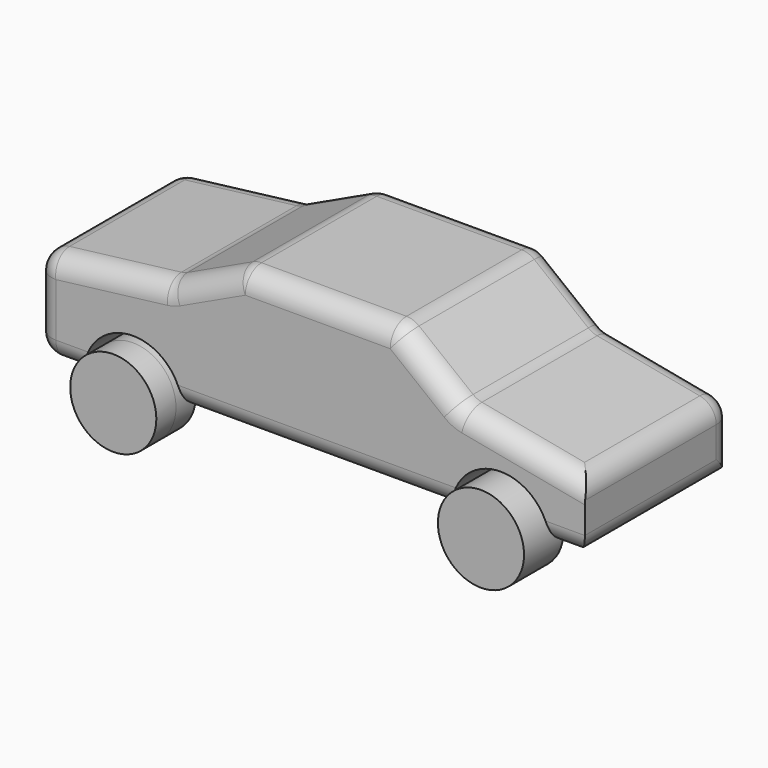
from build123d import *

# Parameters (mm, degrees)
F1_DEPTH     = 19.05
F4_DEPTH     = 12.7
F6_R         = 8.89
F5_R         = 8.89
F7_DEPTH     = 5.08
F8_T1_DEPTH  = 38.1
F8_T3_DEPTH  = 29.9173936093
F8_T5_DEPTH  = 29.718
F8_T7_DEPTH  = 14.8935742204
F8_T9_DEPTH  = 23.2557715278
F8_T11_DEPTH = 14.2243314288
F8_T13_DEPTH = 21.5680204606
F8_T15_DEPTH = 42.5791602327
F8_T17_DEPTH = 35.5135845537
F8_T19_DEPTH = 76.5302014148
F8_T21_DEPTH = 59.055
F8_T23_DEPTH = 28.168599112
F8_T25_DEPTH = 16.2432985797
F8_T27_DEPTH = 10.996646743
F8_T29_DEPTH = 76.2253981626
F8_T31_DEPTH = 16.5481018319
F8_T33_DEPTH = 21.0302364974
F8_T38_DEPTH = 4.27482
F8_T44_DEPTH = 4.27482
F8_T50_DEPTH = 4.27482
F8_T56_DEPTH = 4.27482
F8_T62_DEPTH = 4.27482
F8_T68_DEPTH = 4.27482
F8_T74_DEPTH = 4.27482
F8_S79_W     = 4.27482
F8_S79_H     = 4.27482
F8_T80_DEPTH = 4.27482
F8_S85_W     = 4.27482
F8_S85_H     = 4.27482
F8_T86_DEPTH = 4.27482
F8_T90_ANGLE = 27.5490340182
F8_T92_ANGLE = 18.1765244607
F8_T94_ANGLE = 18.1765244607
F8_T96_ANGLE = 27.5490340182
F9_T         = 2.54
F9_T4_ANGLE  = 180.000000001
F9_T6_ANGLE  = 180.000000001
F9_T8_ANGLE  = 180.000000001
F9_T10_ANGLE = 180.000000001


# Not quite as in the source:
# - a fillet or chamfer that OpenCascade refuses, or shapes differently, is made with other operations: its cross-section is extruded or revolved along the edge and cut away or added
# - a shell that OpenCascade refuses in one call is made with other operations: the cavity is built on its own and cut out


with BuildPart() as f1:
    # F0 (on Front) → F1 (new body, symmetric)
    with BuildSketch(Plane.XZ):
        Polygon((-51.9683994353, 0), (61.4171996713, 0), (61.4171996713, 14.0208005905), (35.8140021563, 18.897600472), (22.7076001465, 29.2607992887), (-9.6011999995, 29.2607992887), (-24.5363991708, 22.2504008561), (-51.9683994353, 18.897600472), (-51.9683994353, 4.5719998889), align=None)
    extrude(amount=F1_DEPTH, both=True)

    # F3 (on face) + F2 (on face) → F4 (cut, symmetric)
    with BuildSketch(Plane.XZ.offset(19.05)):
        with BuildLine():
            Line((-42.0116008556, 0), (-21.6916008556, 0))
            ThreePointArc((-21.6916008556, 0), (-31.8516008556, 10.16), (-42.0116008556, 0))
        make_face()
        with BuildLine():
            Line((54.2036005592, 0), (33.8836005592, 0))
            ThreePointArc((33.8836005592, 0), (44.0436005592, -10.16), (54.2036005592, 0))
        make_face()
        with BuildLine():
            ThreePointArc((54.2036005592, 0), (44.0436005592, 10.16), (33.8836005592, 0))
            Line((33.8836005592, 0), (54.2036005592, 0))
        make_face()
        with BuildLine():
            ThreePointArc((-42.0116008556, 0), (-31.8516008556, -10.16), (-21.6916008556, 0))
            Line((-21.6916008556, 0), (-42.0116008556, 0))
        make_face()
    with BuildSketch(Plane(origin=(0, 19.05, 0), x_dir=(-1, 0, 0), z_dir=(0, 1, 0))):
        with BuildLine():
            ThreePointArc((41.7067976034, 0), (31.5467976034, 10.16), (21.3867976034, 0))
            Line((21.3867976034, 0), (41.7067976034, 0))
        make_face()
        with BuildLine():
            ThreePointArc((-54.2036005592, 0), (-44.0436005592, -10.16), (-33.8836005592, 0))
            Line((-33.8836005592, 0), (-54.2036005592, 0))
        make_face()
        with BuildLine():
            Line((-54.2036005592, 0), (-33.8836005592, 0))
            ThreePointArc((-33.8836005592, 0), (-44.0436005592, 10.16), (-54.2036005592, 0))
        make_face()
        with BuildLine():
            Line((41.7067976034, 0), (21.3867976034, 0))
            ThreePointArc((21.3867976034, 0), (31.5467976034, -10.16), (41.7067976034, 0))
        make_face()
    extrude(amount=F4_DEPTH, both=True, dir=(0, -1, 0), mode=Mode.SUBTRACT)

    # F8: fillet of radius 4.191 on 26 edges, made by hand

    # F8_s2 → F8_t1 (join)
    with BuildSketch(Plane.XZ.offset(-19.05)):
        with BuildLine():
            ThreePointArc((-25.2018560669, 22.169067227), (-24.551136176, 22.3016042151), (-23.9295202845, 22.5352623263))
            Line((-23.9295202845, 22.5352623263), (-24.5363991708, 22.2504008561))
            Line((-24.5363991708, 22.2504008561), (-25.2018560669, 22.169067227))
        make_face()
        with BuildLine():
            ThreePointArc((35.008068319, 19.5348503123), (35.8655819494, 19.0104747998), (36.8232883246, 18.7053554735))
            Line((36.8232883246, 18.7053554735), (35.8140021563, 18.897600472))
            Line((35.8140021563, 18.897600472), (35.008068319, 19.5348503123))
        make_face()
    extrude(amount=F8_T1_DEPTH)

    # F8_s4 → F8_t3 (cut)
    with BuildSketch(Plane.YZ.offset(-8.6665206958)):
        with BuildLine():
            ThreePointArc((-19.05, 25.0697992887), (-17.82248452, 28.0332838087), (-14.859, 29.2607992887))
            Line((-14.859, 29.2607992887), (-19.05, 29.2607992887))
            Line((-19.05, 29.2607992887), (-19.05, 25.0697992887))
        make_face()
        with BuildLine():
            ThreePointArc((19.05, 25.0697992887), (17.82248452, 28.0332838087), (14.859, 29.2607992887))
            Line((14.859, 29.2607992887), (19.05, 29.2607992887))
            Line((19.05, 29.2607992887), (19.05, 25.0697992887))
        make_face()
    extrude(amount=F8_T3_DEPTH, mode=Mode.SUBTRACT)

    # F8_s6 → F8_t5 (cut)
    with BuildSketch(Plane.XZ.offset(-14.859)):
        with BuildLine():
            ThreePointArc((-10.4473062617, 28.8636474365), (-9.5787880395, 29.1603065059), (-8.6665206958, 29.2607992887))
            Line((-8.6665206958, 29.2607992887), (-9.6011999995, 29.2607992887))
            Line((-9.6011999995, 29.2607992887), (-10.4473062617, 28.8636474365))
        make_face()
        with BuildLine():
            ThreePointArc((-51.9683994353, 15.187646743), (-50.9155034841, 17.9655567449), (-48.2858492188, 19.3476899901))
            Line((-48.2858492188, 19.3476899901), (-51.9683994353, 18.897600472))
            Line((-51.9683994353, 18.897600472), (-51.9683994353, 15.187646743))
        make_face()
        with BuildLine():
            ThreePointArc((21.2508729135, 29.2607992887), (22.6268501713, 29.0284818456), (23.8502798184, 28.3572853713))
            Line((23.8502798184, 28.3572853713), (22.7076001465, 29.2607992887))
            Line((22.7076001465, 29.2607992887), (21.2508729135, 29.2607992887))
        make_face()
        with BuildLine():
            ThreePointArc((-47.7773994353, 0), (-50.7408839552, 1.22751548), (-51.9683994353, 4.191))
            Line((-51.9683994353, 4.191), (-51.9683994353, 0))
            Line((-51.9683994353, 0), (-47.7773994353, 0))
        make_face()
    extrude(amount=F8_T5_DEPTH, mode=Mode.SUBTRACT)

    # F8_s8 → F8_t7 (cut)
    with BuildSketch(Plane(origin=(2.5410728022, 0, 1.1927482577), x_dir=(0, 1, 0), z_dir=(-0.9052369715, 0, -0.4249070785))):
        with BuildLine():
            ThreePointArc((-19.05, -26.3765751749), (-17.82248452, -29.3400596948), (-14.859, -30.5675751749))
            Line((-14.859, -30.5675751749), (-19.05, -30.5675751749))
            Line((-19.05, -30.5675751749), (-19.05, -26.3765751749))
        make_face()
        with BuildLine():
            ThreePointArc((19.05, -26.3765751749), (17.82248452, -29.3400596948), (14.859, -30.5675751749))
            Line((14.859, -30.5675751749), (19.05, -30.5675751749))
            Line((19.05, -30.5675751749), (19.05, -26.3765751749))
        make_face()
    extrude(amount=F8_T7_DEPTH, mode=Mode.SUBTRACT)

    # F8_s10 → F8_t9 (cut)
    with BuildSketch(Plane(origin=(-22.1612522468, 0, -2.7085977811), x_dir=(0, 1, 0), z_dir=(-0.9926135164, 0, -0.1213194425))):
        with BuildLine():
            ThreePointArc((19.05, -20.8717909029), (17.82248452, -23.8352754229), (14.859, -25.0627909029))
            Line((14.859, -25.0627909029), (19.05, -25.0627909029))
            Line((19.05, -25.0627909029), (19.05, -20.8717909029))
        make_face()
        with BuildLine():
            ThreePointArc((-19.05, -20.8717909029), (-17.82248452, -23.8352754229), (-14.859, -25.0627909029))
            Line((-14.859, -25.0627909029), (-19.05, -25.0627909029))
            Line((-19.05, -25.0627909029), (-19.05, -20.8717909029))
        make_face()
    extrude(amount=F8_T9_DEPTH, mode=Mode.SUBTRACT)

    # F8_s12 → F8_t11 (cut)
    with BuildSketch(Plane(origin=(12.0365997504, 0, -9.5173088845), x_dir=(0, 1, 0), z_dir=(-0.7844156723, 0, 0.6202354819))):
        with BuildLine():
            ThreePointArc((19.05, -32.8456888666), (17.82248452, -35.8091733865), (14.859, -37.0366888666))
            Line((14.859, -37.0366888666), (19.05, -37.0366888666))
            Line((19.05, -37.0366888666), (19.05, -32.8456888666))
        make_face()
        with BuildLine():
            ThreePointArc((-19.05, -32.8456888666), (-17.82248452, -35.8091733865), (-14.859, -37.0366888666))
            Line((-14.859, -37.0366888666), (-19.05, -37.0366888666))
            Line((-19.05, -37.0366888666), (-19.05, -32.8456888666))
        make_face()
    extrude(amount=F8_T11_DEPTH, mode=Mode.SUBTRACT)

    # F8_s14 → F8_t13 (cut)
    with BuildSketch(Plane(origin=(53.2829846843, 0, -10.1491406782), x_dir=(0, 1, 0), z_dir=(-0.9823385639, 0, 0.187112121))):
        with BuildLine():
            ThreePointArc((19.05, -21.0740756151), (17.82248452, -24.037560135), (14.859, -25.2650756151))
            Line((14.859, -25.2650756151), (19.05, -25.2650756151))
            Line((19.05, -25.2650756151), (19.05, -21.0740756151))
        make_face()
    extrude(amount=F8_T13_DEPTH, mode=Mode.SUBTRACT)

    # F8_s16 → F8_t15 (cut)
    with BuildSketch(Plane.XZ.offset(-14.859)):
        with BuildLine():
            ThreePointArc((61.4171996713, 10.5527364974), (60.4550545995, 13.2246228821), (58.0103865705, 14.6697174188))
            Line((58.0103865705, 14.6697174188), (61.4171996713, 14.0208005905))
            Line((61.4171996713, 14.0208005905), (61.4171996713, 10.5527364974))
        make_face()
    extrude(amount=F8_T15_DEPTH, mode=Mode.SUBTRACT)

    # F8_s18 → F8_t17 (cut)
    with BuildSketch(Plane(origin=(66.9822500885, 0, -12.7585247546), x_dir=(0, 1, 0), z_dir=(-0.9823385639, 0, 0.187112121))):
        with BuildLine():
            ThreePointArc((-19.05, -21.0740756151), (-17.82248452, -24.037560135), (-14.859, -25.2650756151))
            Line((-14.859, -25.2650756151), (-19.05, -25.2650756151))
            Line((-19.05, -25.2650756151), (-19.05, -21.0740756151))
        make_face()
    extrude(amount=F8_T17_DEPTH, mode=Mode.SUBTRACT)

    # F8_s20 → F8_t19 (cut)
    with BuildSketch(Plane.YZ.offset(-32.1691008556)):
        with BuildLine():
            ThreePointArc((-14.859, 0), (-17.82248452, 1.22751548), (-19.05, 4.191))
            Line((-19.05, 4.191), (-19.05, 0))
            Line((-19.05, 0), (-14.859, 0))
        make_face()
    extrude(amount=F8_T19_DEPTH, mode=Mode.SUBTRACT)

    # F8_s22 → F8_t21 (cut)
    with BuildSketch(Plane.XZ.offset(-29.5275)):
        with BuildLine():
            ThreePointArc((57.2261996713, 0), (60.1896841912, 1.22751548), (61.4171996713, 4.191))
            Line((61.4171996713, 4.191), (61.4171996713, 0))
            Line((61.4171996713, 0), (57.2261996713, 0))
        make_face()
    extrude(amount=F8_T21_DEPTH, mode=Mode.SUBTRACT)

    # F8_s24 → F8_t23 (cut)
    with BuildSketch(Plane.YZ.offset(43.7261005592)):
        with BuildLine():
            ThreePointArc((-14.859, 0), (-17.82248452, 1.22751548), (-19.05, 4.191))
            Line((-19.05, 4.191), (-19.05, 0))
            Line((-19.05, 0), (-14.859, 0))
        make_face()
    extrude(amount=F8_T23_DEPTH, mode=Mode.SUBTRACT)

    # F8_s26 → F8_t25 (cut)
    with BuildSketch(Plane.YZ.offset(-47.7773994353)):
        with BuildLine():
            ThreePointArc((-14.859, 0), (-17.82248452, 1.22751548), (-19.05, 4.191))
            Line((-19.05, 4.191), (-19.05, 0))
            Line((-19.05, 0), (-14.859, 0))
        make_face()
    extrude(amount=F8_T25_DEPTH, mode=Mode.SUBTRACT)

    # F8_s28 → F8_t27 (cut)
    with BuildSketch(Plane.XY.offset(4.191)):
        with BuildLine():
            ThreePointArc((-47.7773994353, 19.05), (-50.7408839552, 17.82248452), (-51.9683994353, 14.859))
            Line((-51.9683994353, 14.859), (-51.9683994353, 19.05))
            Line((-51.9683994353, 19.05), (-47.7773994353, 19.05))
        make_face()
        with BuildLine():
            ThreePointArc((-51.9683994353, -14.859), (-50.7408839552, -17.82248452), (-47.7773994353, -19.05))
            Line((-47.7773994353, -19.05), (-51.9683994353, -19.05))
            Line((-51.9683994353, -19.05), (-51.9683994353, -14.859))
        make_face()
    extrude(amount=F8_T27_DEPTH, mode=Mode.SUBTRACT)

    # F8_s30 → F8_t29 (cut)
    with BuildSketch(Plane.YZ.offset(-31.8642976034)):
        with BuildLine():
            ThreePointArc((14.859, 0), (17.82248452, 1.22751548), (19.05, 4.191))
            Line((19.05, 4.191), (19.05, 0))
            Line((19.05, 0), (14.859, 0))
        make_face()
    extrude(amount=F8_T29_DEPTH, mode=Mode.SUBTRACT)

    # F8_s32 → F8_t31 (cut)
    with BuildSketch(Plane.YZ.offset(-47.7773994353)):
        with BuildLine():
            ThreePointArc((14.859, 0), (17.82248452, 1.22751548), (19.05, 4.191))
            Line((19.05, 4.191), (19.05, 0))
            Line((19.05, 0), (14.859, 0))
        make_face()
    extrude(amount=F8_T31_DEPTH, mode=Mode.SUBTRACT)

    # F8_s34 → F8_t33 (cut)
    with BuildSketch(Plane.XY.offset(-10.4775)):
        with BuildLine():
            ThreePointArc((57.2261996713, 19.05), (60.1896841912, 17.82248452), (61.4171996713, 14.859))
            Line((61.4171996713, 14.859), (61.4171996713, 19.05))
            Line((61.4171996713, 19.05), (57.2261996713, 19.05))
        make_face()
    extrude(amount=F8_T33_DEPTH, mode=Mode.SUBTRACT)


with BuildPart() as f7:
    # F6 (on face) + F5 (on face) → F7 (new body, symmetric)
    with BuildSketch(Plane(origin=(0, 19.05, 0), x_dir=(-1, 0, 0), z_dir=(0, 1, 0))):
        with Locations((-44.0436005592, 0)):
            Circle(F6_R)
        with Locations((31.5467976034, 0)):
            Circle(F6_R)
    with BuildSketch(Plane.XZ.offset(19.05)):
        with Locations((44.0436005592, 0)):
            Circle(F5_R)
        with Locations((-31.8516008556, 0)):
            Circle(F5_R)
    extrude(amount=F7_DEPTH, both=True, dir=(0, 1, 0))


with BuildPart() as f8_tool36:
    # F8_s37 → F8_t38 (new body)
    with BuildSketch(Plane.XZ.offset(14.859)):
        Polygon((21.2508729135, 25.0697992887), (21.2508729135, 29.3446192887), (22.7367346912, 29.3446192887), (23.9022679564, 28.423035093), align=None)
    extrude(amount=F8_T38_DEPTH)

    # F8_s39 → F8_t40 (revolve, cut)
    with BuildSketch(Plane(origin=(21.2508729135, -14.859, 25.0697992887), x_dir=(-0.3283171696, 0, -0.9445675392), z_dir=(-0.9445675392, 0, 0.3283171696))):
        with BuildLine():
            ThreePointArc((0, -4.191), (4.191, 0), (0, 4.191))
            Line((0, 4.191), (0, -4.191))
        make_face()
    revolve(axis=Axis((21.2508729135, -14.859, 25.0697992887), (0, -1, 0)), mode=Mode.SUBTRACT)


with BuildPart() as f1_1:
    add(f1.part)

    # F8_t35: cut F8_tool36
    add(f8_tool36.part, mode=Mode.SUBTRACT)


with BuildPart() as f8_tool42:
    # F8_s43 → F8_t44 (new body)
    with BuildSketch(Plane.XZ.offset(14.859)):
        Polygon((-8.6665206958, 25.0697992887), (-10.482921973, 28.9395243995), (-9.6198935855, 29.3446192887), (-8.6665206958, 29.3446192887), align=None)
    extrude(amount=F8_T44_DEPTH)

    # F8_s45 → F8_t46 (revolve, cut)
    with BuildSketch(Plane(origin=(-8.6665206958, -14.859, 25.0697992887), x_dir=(0.2176729524, 0, -0.976021765), z_dir=(-0.976021765, 0, -0.2176729524))):
        with BuildLine():
            ThreePointArc((0, -4.191), (4.191, 0), (0, 4.191))
            Line((0, 4.191), (0, -4.191))
        make_face()
    revolve(axis=Axis((-8.6665206958, -14.859, 25.0697992887), (0, -1, 0)), mode=Mode.SUBTRACT)


with BuildPart() as f1_2:
    add(f1_1.part)

    # F8_t41: cut F8_tool42
    add(f8_tool42.part, mode=Mode.SUBTRACT)


with BuildPart() as f8_tool48:
    # F8_s49 → F8_t50 (new body)
    with BuildSketch(Plane.XZ.offset(-14.859)):
        Polygon((-8.6665206958, 25.0697992887), (-10.482921973, 28.9395243995), (-9.6198935855, 29.3446192887), (-8.6665206958, 29.3446192887), align=None)
    extrude(amount=-F8_T50_DEPTH)

    # F8_s51 → F8_t52 (revolve, cut)
    with BuildSketch(Plane(origin=(-8.6665206958, 14.859, 25.0697992887), x_dir=(0.2176729524, 0, -0.976021765), z_dir=(0.976021765, 0, 0.2176729524))):
        with BuildLine():
            ThreePointArc((0, -4.191), (4.191, 0), (0, 4.191))
            Line((0, 4.191), (0, -4.191))
        make_face()
    revolve(axis=Axis((-8.6665206958, 14.859, 25.0697992887), (0, 1, 0)), mode=Mode.SUBTRACT)


with BuildPart() as f1_3:
    add(f1_2.part)

    # F8_t47: cut F8_tool48
    add(f8_tool48.part, mode=Mode.SUBTRACT)


with BuildPart() as f8_tool54:
    # F8_s55 → F8_t56 (new body)
    with BuildSketch(Plane.XZ.offset(14.859)):
        Polygon((-47.7773994353, 15.187646743), (-52.0522194353, 15.187646743), (-52.0522194353, 18.9717995466), (-48.2960182145, 19.430890855), align=None)
    extrude(amount=F8_T56_DEPTH)

    # F8_s57 → F8_t58 (revolve, cut)
    with BuildSketch(Plane(origin=(-47.7773994353, -14.859, 15.187646743), x_dir=(0.7487721424, 0, -0.6628274879), z_dir=(-0.6628274879, 0, -0.7487721424))):
        with BuildLine():
            ThreePointArc((0, -4.191), (4.191, 0), (0, 4.191))
            Line((0, 4.191), (0, -4.191))
        make_face()
    revolve(axis=Axis((-47.7773994353, -14.859, 15.187646743), (0, -1, 0)), mode=Mode.SUBTRACT)


with BuildPart() as f1_4:
    add(f1_3.part)

    # F8_t53: cut F8_tool54
    add(f8_tool54.part, mode=Mode.SUBTRACT)


with BuildPart() as f8_tool60:
    # F8_s61 → F8_t62 (new body)
    with BuildSketch(Plane.XZ.offset(-14.859)):
        Polygon((-47.7773994353, 15.187646743), (-52.0522194353, 15.187646743), (-52.0522194353, 18.9717995466), (-48.2960182145, 19.430890855), align=None)
    extrude(amount=-F8_T62_DEPTH)

    # F8_s63 → F8_t64 (revolve, cut)
    with BuildSketch(Plane(origin=(-47.7773994353, 14.859, 15.187646743), x_dir=(0.7487721424, 0, -0.6628274879), z_dir=(0.6628274879, 0, 0.7487721424))):
        with BuildLine():
            ThreePointArc((0, -4.191), (4.191, 0), (0, 4.191))
            Line((0, 4.191), (0, -4.191))
        make_face()
    revolve(axis=Axis((-47.7773994353, 14.859, 15.187646743), (0, 1, 0)), mode=Mode.SUBTRACT)


with BuildPart() as f1_5:
    add(f1_4.part)

    # F8_t59: cut F8_tool60
    add(f8_tool60.part, mode=Mode.SUBTRACT)


with BuildPart() as f8_tool66:
    # F8_s67 → F8_t68 (new body)
    with BuildSketch(Plane.XZ.offset(-14.859)):
        Polygon((21.2508729135, 25.0697992887), (21.2508729135, 29.3446192887), (22.7367346912, 29.3446192887), (23.9022679564, 28.423035093), align=None)
    extrude(amount=-F8_T68_DEPTH)

    # F8_s69 → F8_t70 (revolve, cut)
    with BuildSketch(Plane(origin=(21.2508729135, 14.859, 25.0697992887), x_dir=(-0.3283171696, 0, -0.9445675392), z_dir=(0.9445675392, 0, -0.3283171696))):
        with BuildLine():
            ThreePointArc((0, -4.191), (4.191, 0), (0, 4.191))
            Line((0, 4.191), (0, -4.191))
        make_face()
    revolve(axis=Axis((21.2508729135, 14.859, 25.0697992887), (0, 1, 0)), mode=Mode.SUBTRACT)


with BuildPart() as f1_6:
    add(f1_5.part)

    # F8_t65: cut F8_tool66
    add(f8_tool66.part, mode=Mode.SUBTRACT)


with BuildPart() as f8_tool72:
    # F8_s73 → F8_t74 (new body)
    with BuildSketch(Plane.XZ.offset(-14.859)):
        Polygon((57.2261996713, 10.5527364974), (58.0260703085, 14.7520570373), (61.5010196713, 14.0901618724), (61.5010196713, 10.5527364974), align=None)
    extrude(amount=-F8_T74_DEPTH)

    # F8_s75 → F8_t76 (revolve, cut)
    with BuildSketch(Plane(origin=(57.2261996713, 14.859, 10.5527364974), x_dir=(-0.7704258955, 0, -0.6375295597), z_dir=(0.6375295597, 0, -0.7704258955))):
        with BuildLine():
            ThreePointArc((0, -4.191), (4.191, 0), (0, 4.191))
            Line((0, 4.191), (0, -4.191))
        make_face()
    revolve(axis=Axis((57.2261996713, 14.859, 10.5527364974), (0, 1, 0)), mode=Mode.SUBTRACT)


with BuildPart() as f1_7:
    add(f1_6.part)

    # F8_t71: cut F8_tool72
    add(f8_tool72.part, mode=Mode.SUBTRACT)


with BuildPart() as f8_tool78:
    # F8_s79 → F8_t80 (new body)
    with BuildSketch(Plane.XY.offset(4.191)):
        with Locations((-49.9148094353, -16.99641)):
            Rectangle(F8_S79_W, F8_S79_H)
    extrude(amount=-F8_T80_DEPTH)

    # F8_s81 → F8_t82 (revolve, cut)
    with BuildSketch(Plane(origin=(-47.7773994353, -14.859, 4.191), x_dir=(0.7071067812, 0.7071067812, 0), z_dir=(-0.7071067812, 0.7071067812, 0))):
        with BuildLine():
            ThreePointArc((0, -4.191), (4.191, 0), (0, 4.191))
            Line((0, 4.191), (0, -4.191))
        make_face()
    revolve(axis=Axis((-47.7773994353, -14.859, 4.191), (0, 0, -1)), mode=Mode.SUBTRACT)


with BuildPart() as f1_8:
    add(f1_7.part)

    # F8_t77: cut F8_tool78
    add(f8_tool78.part, mode=Mode.SUBTRACT)


with BuildPart() as f8_tool84:
    # F8_s85 → F8_t86 (new body)
    with BuildSketch(Plane.XY.offset(4.191)):
        with Locations((-49.9148094353, 16.99641)):
            Rectangle(F8_S85_W, F8_S85_H)
    extrude(amount=-F8_T86_DEPTH)

    # F8_s87 → F8_t88 (revolve, cut)
    with BuildSketch(Plane(origin=(-47.7773994353, 14.859, 4.191), x_dir=(0.7071067812, -0.7071067812, 0), z_dir=(0.7071067812, 0.7071067812, 0))):
        with BuildLine():
            ThreePointArc((0, -4.191), (4.191, 0), (0, 4.191))
            Line((0, 4.191), (0, -4.191))
        make_face()
    revolve(axis=Axis((-47.7773994353, 14.859, 4.191), (0, 0, -1)), mode=Mode.SUBTRACT)


with BuildPart() as f1_9:
    add(f1_8.part)

    # F8_t83: cut F8_tool84
    add(f8_tool84.part, mode=Mode.SUBTRACT)

    # F8_s89 → F8_t90 (revolve, cut)
    with BuildSketch(Plane(origin=(12.0365997504, 0, -9.5173088845), x_dir=(0, 1, 0), z_dir=(-0.7844156723, 0, 0.6202354819))):
        with BuildLine():
            ThreePointArc((-19.05, -32.8456888666), (-17.82248452, -35.8091733865), (-14.859, -37.0366888666))
            Line((-14.859, -37.0366888666), (-19.05, -37.0366888666))
            Line((-19.05, -37.0366888666), (-19.05, -32.8456888666))
        make_face()
    revolve(axis=Axis((37.6074752238, -19.05, 22.8223363949), (0, -1, 0)), revolution_arc=F8_T90_ANGLE, mode=Mode.SUBTRACT)

    # F8_s91 → F8_t92 (revolve, cut)
    with BuildSketch(Plane(origin=(-22.1612522468, 0, -2.7085977811), x_dir=(0, 1, 0), z_dir=(-0.9926135164, 0, -0.1213194425))):
        with BuildLine():
            ThreePointArc((-19.05, -20.8717909029), (-17.82248452, -23.8352754229), (-14.859, -25.0627909029))
            Line((-14.859, -25.0627909029), (-19.05, -25.0627909029))
            Line((-19.05, -25.0627909029), (-19.05, -20.8717909029))
        make_face()
    revolve(axis=Axis((-25.7103058504, -19.05, 26.3291104741), (0, -1, 0)), revolution_arc=F8_T92_ANGLE, mode=Mode.SUBTRACT)

    # F8_s93 → F8_t94 (revolve, cut)
    with BuildSketch(Plane(origin=(-22.1612522468, 0, -2.7085977811), x_dir=(0, 1, 0), z_dir=(-0.9926135164, 0, -0.1213194425))):
        with BuildLine():
            ThreePointArc((19.05, -20.8717909029), (17.82248452, -23.8352754229), (14.859, -25.0627909029))
            Line((14.859, -25.0627909029), (19.05, -25.0627909029))
            Line((19.05, -25.0627909029), (19.05, -20.8717909029))
        make_face()
    revolve(axis=Axis((-25.7103058504, 19.05, 26.3291104741), (0, -1, 0)), revolution_arc=F8_T94_ANGLE, mode=Mode.SUBTRACT)

    # F8_s95 → F8_t96 (revolve, cut)
    with BuildSketch(Plane(origin=(12.0365997504, 0, -9.5173088845), x_dir=(0, 1, 0), z_dir=(-0.7844156723, 0, 0.6202354819))):
        with BuildLine():
            ThreePointArc((19.05, -32.8456888666), (17.82248452, -35.8091733865), (14.859, -37.0366888666))
            Line((14.859, -37.0366888666), (19.05, -37.0366888666))
            Line((19.05, -37.0366888666), (19.05, -32.8456888666))
        make_face()
    revolve(axis=Axis((37.6074752238, 19.05, 22.8223363949), (0, -1, 0)), revolution_arc=F8_T96_ANGLE, mode=Mode.SUBTRACT)

    # F9: shell of thickness 2.54, made by hand


with BuildPart() as f9_core1:
    # F9_t2: copy of F1
    add(f1_9.part)

    # the walls: a layer under each face that stays
    f9_faces = [f9_core1.faces().sort_by_distance(p)[0] for p in [
        (-31.5467976034, 12.7, 10.16),
        (-31.5467976034, 6.35, 5.08),
        (-44.2897631301, 17.82248452, 1.22751548),
        (-50.7408839552, 0, 1.2275154801),
        (-44.4421647562, -17.82248452, 1.22751548),
        (-31.8516008556, -12.7, 10.16),
        (-31.8516008556, -6.35, 5.08),
        (6.0959998518, -17.82248452, 1.22751548),
        (44.0436005592, -12.7, 10.16),
        (44.0436005592, -6.35, 5.08),
        (57.358064726, -17.82248452, 1.22751548),
        (60.1896841913, 0, 1.2275154801),
        (4.724400118, 19.05, 12.5348996444),
        (44.0436005592, 12.7, 10.16),
        (44.0436005592, 6.35, 5.08),
        (6.2484014779, 17.82248452, 1.22751548),
        (-49.8728994354, 16.9545000001, 1.2275154802),
        (-51.9683994353, 0, 9.6893233715),
        (-49.8728994354, -16.9545000001, 1.2275154802),
        (6.819900118, -19.05, 14.6303996444),
        (61.4171996713, -2.0955, 7.3718682487),
        (60.1896841913, 17.8224845199, 5.2763682487),
        (-24.2116232389, 17.82248452, 21.1219749432),
        (-16.6668332567, 17.8224845199, 24.5882624857),
        (6.2921761089, 17.82248452, 28.0332838087),
        (28.6678254133, 17.8224845199, 22.9831854613),
        (35.3553932214, 17.8224845199, 17.8940063876),
        (47.1871544225, 17.8224845199, 15.4817006524),
        (-50.7408839552, 17.8224845199, 9.6893233715),
        (-36.5949311491, 17.82248452, 19.5399301515),
        (-50.9155034841, 0, 17.9655567449),
        (-50.7408839552, -17.8224845199, 9.6893233715),
        (-36.5949311491, -17.82248452, 19.5399301515),
        (-24.2116232389, -17.82248452, 21.1219749432),
        (-16.6668332567, -17.8224845199, 24.5882624857),
        (6.2921761089, -17.82248452, 28.0332838087),
        (28.6678254133, -17.8224845199, 22.9831854613),
        (35.3553932214, -17.8224845199, 17.8940063876),
        (49.2826544225, -17.8224845199, 15.0825577662),
        (60.4550545995, -2.0584904607, 13.2246228821),
        (59.5093448865, 17.82248452, 12.4420454786),
        (-24.551136176, 0, 22.3016042151),
        (-17.1884132731, 0, 25.6994548814),
        (-9.3115911206, 17.8224845198, 27.9622246806),
        (6.2921761089, 0, 29.2607992887),
        (22.2238357633, 17.8224845198, 27.8690105694),
        (29.4291740687, 0, 23.9460678418),
        (35.8655819494, 0, 19.0104747998),
        (47.4168374476, 0, 16.6875364462),
        (-49.9963740884, 17.8224845198, 17.151925743),
        (-36.7438526428, 0, 20.7583786085),
        (-49.9963740884, -17.8224845198, 17.151925743),
        (-9.3115911206, -17.8224845198, 27.9622246806),
        (22.2238357633, -17.8224845198, 27.8690105694),
        (-9.5787880395, 0, 29.1603065059),
        (22.6268501713, 0, 29.0284818456),
    ]]
    thicken(f9_faces, amount=-F9_T, mode=Mode.SUBTRACT)

    # F9_s3 → F9_t4 (revolve, cut)
    with BuildSketch(Plane.XY):
        Polygon((-41.6813976034, 6.3754), (-44.2467976034, 6.35), (-44.2467976034, 3.81), (-41.7067976034, 3.81), align=None)
    revolve(axis=Axis((-31.5467976034, 6.35, 0), (0, 1, 0)), revolution_arc=F9_T4_ANGLE, mode=Mode.SUBTRACT)

    # F9_s5 → F9_t6 (revolve, cut)
    with BuildSketch(Plane.XY):
        Polygon((-21.7170008556, -6.3754), (-19.1516008556, -6.35), (-19.1516008556, -3.81), (-21.6916008556, -3.81), align=None)
    revolve(axis=Axis((-31.8516008556, -6.35, 0), (0, -1, 0)), revolution_arc=F9_T6_ANGLE, mode=Mode.SUBTRACT)

    # F9_s7 → F9_t8 (revolve, cut)
    with BuildSketch(Plane.XY):
        Polygon((54.1782005592, -6.3754), (56.7436005592, -6.35), (56.7436005592, -3.81), (54.2036005592, -3.81), align=None)
    revolve(axis=Axis((44.0436005592, -6.35, 0), (0, -1, 0)), revolution_arc=F9_T8_ANGLE, mode=Mode.SUBTRACT)

    # F9_s9 → F9_t10 (revolve, cut)
    with BuildSketch(Plane.XY):
        Polygon((33.9090005592, 6.3754), (31.3436005592, 6.35), (31.3436005592, 3.81), (33.8836005592, 3.81), align=None)
    revolve(axis=Axis((44.0436005592, 6.35, 0), (0, 1, 0)), revolution_arc=F9_T10_ANGLE, mode=Mode.SUBTRACT)


with BuildPart() as f1_10:
    add(f1_9.part)

    # what is left inside the walls is the cavity
    f9_cavity = [f9_core1.part.solids().sort_by_distance(p)[0] for p in [
        (4.7244, 6.053667, 0.0254),
    ]]
    add(f9_cavity, mode=Mode.SUBTRACT)


solid = Compound([f7.part, f1_10.part])
